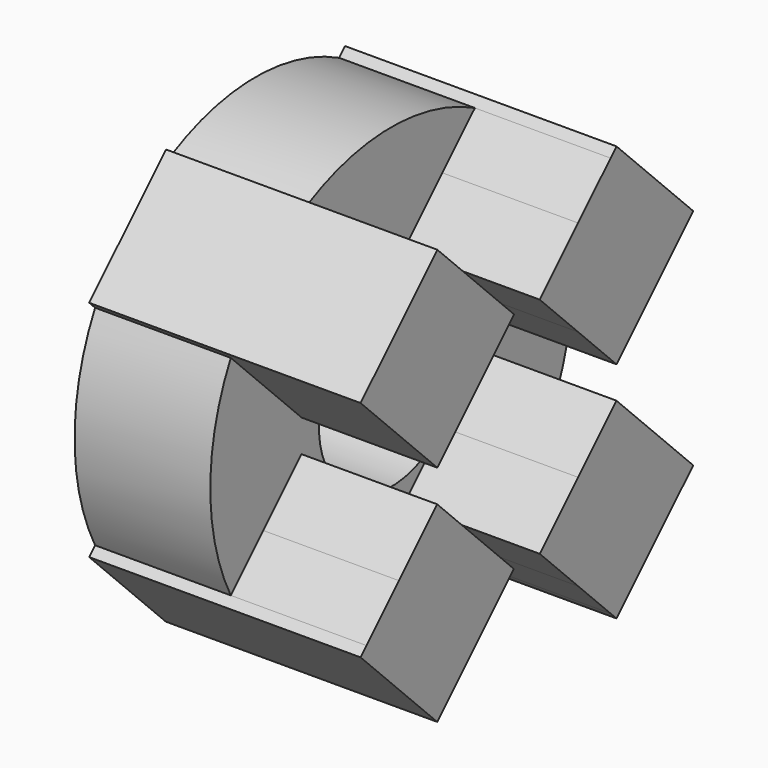
from build123d import *

# Parameters (mm, degrees)
F1_DEPTH = 7.62
F2_DEPTH = 15.24


with BuildPart() as f1:
    # F0 (on Right) → F1 (new body)
    with BuildSketch(Plane.YZ):
        with BuildLine():
            ThreePointArc((-22.7695842606, 19.3196809519), (-21.6955753206, 22.1687878641), (-21.330579045, 25.1916479534))
            ThreePointArc((-21.330579045, 25.1916479534), (-21.6955753206, 28.2145080427), (-22.7695842606, 31.063614955))
            Line((-22.7695842606, 31.063614955), (-25.0498647737, 28.7835671044))
            Line((-25.0498647737, 28.7835671044), (-25.0498647737, 21.5997288025))
            Line((-25.0498647737, 21.5997288025), (-22.7695842606, 19.3196809519))
        make_face()
        with BuildLine():
            Line((-25.0498647737, 28.7835671044), (-22.7695842606, 31.063614955))
            ThreePointArc((-22.7695842606, 31.063614955), (-23.7911283922, 32.7045468833), (-25.0498647737, 34.1714459009))
            Line((-25.0498647737, 34.1714459009), (-25.0498647737, 28.7835671044))
        make_face()
        with BuildLine():
            ThreePointArc((-24.8535283353, 16.4125967363), (-23.7086988595, 17.7924054626), (-22.7695842606, 19.3196809519))
            Line((-22.7695842606, 19.3196809519), (-25.0498647737, 21.5997288025))
            Line((-25.0498647737, 21.5997288025), (-25.0498647737, 16.2165853811))
            Line((-25.0498647737, 16.2165853811), (-24.8535283353, 16.4125967363))
        make_face()
        with BuildLine():
            Line((-30.4382933645, 34.1714459009), (-25.0498647737, 34.1714459009))
            ThreePointArc((-25.0498647737, 34.1714459009), (-26.5166353453, 35.4303319547), (-28.1574630291, 36.4520435177))
            Line((-28.1574630291, 36.4520435177), (-30.4382933645, 34.1714459009))
        make_face()
        Polygon((-25.0498647737, 28.7835671044), (-25.0498647737, 34.1714459009), (-30.4382933645, 34.1714459009), (-33.1322327207, 31.4777814138), (-30.4382933285, 28.7835671244), (-27.7443539522, 26.089352851), align=None)
        with BuildLine():
            Line((-25.0498647737, 21.5997288025), (-25.0498647737, 28.7835671044))
            Line((-25.0498647737, 28.7835671044), (-27.7443539522, 26.089352851))
            Line((-27.7443539522, 26.089352851), (-30.4382933285, 28.7835671244))
            ThreePointArc((-30.4382933285, 28.7835671244), (-29.3372214281, 27.1355600605), (-28.950579045, 25.1916479534))
            ThreePointArc((-28.950579045, 25.1916479534), (-29.3372214494, 23.2477357949), (-30.4382934071, 21.5997287037))
            Line((-30.4382934071, 21.5997287037), (-27.7443539522, 24.2939430558))
            Line((-27.7443539522, 24.2939430558), (-25.0498647737, 21.5997288025))
        make_face()
        Polygon((-25.0498647737, 16.2165853811), (-25.0498647737, 21.5997288025), (-27.7443539522, 24.2939430558), (-30.4382934071, 21.5997287037), (-33.1280466566, 18.9097009843), (-30.4299203819, 16.2118500059), (-25.0546080025, 16.2118500059), align=None)
        with BuildLine():
            Line((-30.4382933645, 34.1714459009), (-28.1574630291, 36.4520435177))
            ThreePointArc((-28.1574630291, 36.4520435177), (-34.0306965605, 37.8916479529), (-39.9039034491, 36.4519348256))
            Line((-39.9039034491, 36.4519348256), (-37.6234145244, 34.1714459009))
            Line((-37.6234145244, 34.1714459009), (-30.4382933645, 34.1714459009))
        make_face()
        with BuildLine():
            Line((-33.1322327207, 31.4777814138), (-30.4382933645, 34.1714459009))
            Line((-30.4382933645, 34.1714459009), (-37.6234145244, 34.1714459009))
            Line((-37.6234145244, 34.1714459009), (-34.9292002593, 31.4772316359))
            Line((-34.9292002593, 31.4772316359), (-37.6226815049, 28.7837503904))
            ThreePointArc((-37.6226815049, 28.7837503904), (-34.0304494597, 30.2716479518), (-30.4382933285, 28.7835671244))
            Line((-30.4382933285, 28.7835671244), (-33.1322327207, 31.4777814138))
        make_face()
        with BuildLine():
            Line((-37.6234145244, 34.1714459009), (-39.9039034491, 36.4519348256))
            ThreePointArc((-39.9039034491, 36.4519348256), (-41.5446174849, 35.4302624263), (-43.0112933162, 34.1714459009))
            Line((-43.0112933162, 34.1714459009), (-37.6234145244, 34.1714459009))
        make_face()
        Polygon((-34.9292002593, 31.4772316359), (-37.6234145244, 34.1714459009), (-43.0112933162, 34.1714459009), (-43.0112933162, 28.7830173475), (-40.317353932, 26.0890779633), (-37.6226815049, 28.7837503904), align=None)
        with BuildLine():
            ThreePointArc((-28.1519614983, 13.9341235479), (-26.6368414576, 14.865823798), (-25.2667473216, 16.0000619355))
            Line((-25.2667473216, 16.0000619355), (-25.0546080025, 16.2118500059))
            Line((-25.0546080025, 16.2118500059), (-30.4299203819, 16.2118500059))
            Line((-30.4299203819, 16.2118500059), (-28.1519614983, 13.9341235479))
        make_face()
        with BuildLine():
            Line((-33.1280466566, 18.9097009843), (-30.4382934071, 21.5997287037))
            ThreePointArc((-30.4382934071, 21.5997287037), (-37.6225898895, 21.5994539034), (-37.6226815049, 28.7837503904))
            Line((-37.6226815049, 28.7837503904), (-40.317353932, 26.0890779633))
            Line((-40.317353932, 26.0890779633), (-43.0112933162, 28.7830173475))
            Line((-43.0112933162, 28.7830173475), (-43.0112933162, 21.6024270559))
            Line((-43.0112933162, 21.6024270559), (-40.3278979877, 24.2860962057))
            Line((-40.3278979877, 24.2860962057), (-34.9473170757, 18.9060642873))
            Line((-34.9473170757, 18.9060642873), (-37.64125646, 16.2118500059))
            Line((-37.64125646, 16.2118500059), (-30.4299203819, 16.2118500059))
            Line((-30.4299203819, 16.2118500059), (-33.1280466566, 18.9097009843))
        make_face()
        with BuildLine():
            Line((-43.0112933162, 28.7830173475), (-43.0112933162, 34.1714459009))
            ThreePointArc((-43.0112933162, 34.1714459009), (-44.2700992213, 32.7044521275), (-45.2916825052, 31.0634065365))
            Line((-45.2916825052, 31.0634065365), (-43.0112933162, 28.7830173475))
        make_face()
        with BuildLine():
            ThreePointArc((-39.9154717637, 13.9374026349), (-34.034119179, 12.4916484468), (-28.1519614983, 13.9341235479))
            Line((-28.1519614983, 13.9341235479), (-30.4299203819, 16.2118500059))
            Line((-30.4299203819, 16.2118500059), (-37.64125646, 16.2118500059))
            Line((-37.64125646, 16.2118500059), (-39.9154717637, 13.9374026349))
        make_face()
        with BuildLine():
            Line((-43.0112933162, 28.7830173475), (-45.2916825052, 31.0634065365))
            ThreePointArc((-45.2916825052, 31.0634065365), (-46.7305790251, 25.1923579991), (-45.2923390044, 19.3211486035))
            Line((-45.2923390044, 19.3211486035), (-43.0112933162, 21.6024270559))
            Line((-43.0112933162, 21.6024270559), (-43.0112933162, 28.7830173475))
        make_face()
        with BuildLine():
            Line((-40.3262748881, 13.526557591), (-39.9154717637, 13.9374026349))
            ThreePointArc((-39.9154717637, 13.9374026349), (-41.5498772506, 14.9568956607), (-43.0112933162, 16.2118500059))
            ThreePointArc((-43.0112933162, 16.2118500059), (-44.2705192395, 17.6794162735), (-45.2923390044, 19.3211486035))
            Line((-45.2923390044, 19.3211486035), (-45.7073809685, 18.9060642873))
            Line((-45.7073809685, 18.9060642873), (-40.3262748881, 13.526557591))
        make_face()
        with BuildLine():
            ThreePointArc((-43.0112933162, 16.2118500059), (-41.5498772506, 14.9568956607), (-39.9154717637, 13.9374026349))
            Line((-39.9154717637, 13.9374026349), (-37.64125646, 16.2118500059))
            Line((-37.64125646, 16.2118500059), (-43.0112933162, 16.2118500059))
        make_face()
        Polygon((-43.0112933162, 16.2118500059), (-37.64125646, 16.2118500059), (-34.9473170757, 18.9060642873), (-40.3278979877, 24.2860962057), (-43.0112933162, 21.6024270559), align=None)
        with BuildLine():
            Line((-43.0112933162, 21.6024270559), (-45.2923390044, 19.3211486035))
            ThreePointArc((-45.2923390044, 19.3211486035), (-44.2705192395, 17.6794162735), (-43.0112933162, 16.2118500059))
            Line((-43.0112933162, 16.2118500059), (-43.0112933162, 21.6024270559))
        make_face()
    extrude(amount=F1_DEPTH)

    # F0 (on Right) → F2 (join)
    with BuildSketch(Plane.YZ):
        with BuildLine():
            Line((-25.0498647737, 28.7835671044), (-22.7695842606, 31.063614955))
            ThreePointArc((-22.7695842606, 31.063614955), (-23.7911283922, 32.7045468833), (-25.0498647737, 34.1714459009))
            Line((-25.0498647737, 34.1714459009), (-25.0498647737, 28.7835671044))
        make_face()
        with BuildLine():
            ThreePointArc((-25.0498647737, 34.1714459009), (-23.7911283922, 32.7045468833), (-22.7695842606, 31.063614955))
            Line((-22.7695842606, 31.063614955), (-22.3559253895, 31.4772316195))
            Line((-22.3559253895, 31.4772316195), (-25.0498647737, 34.1714459009))
        make_face()
        with BuildLine():
            Line((-22.3559253895, 18.9060642873), (-22.7695842606, 19.3196809519))
            ThreePointArc((-22.7695842606, 19.3196809519), (-23.7086988595, 17.7924054626), (-24.8535283353, 16.4125967363))
            Line((-24.8535283353, 16.4125967363), (-22.3559253895, 18.9060642873))
        make_face()
        with BuildLine():
            ThreePointArc((-24.8535283353, 16.4125967363), (-23.7086988595, 17.7924054626), (-22.7695842606, 19.3196809519))
            Line((-22.7695842606, 19.3196809519), (-25.0498647737, 21.5997288025))
            Line((-25.0498647737, 21.5997288025), (-25.0498647737, 16.2165853811))
            Line((-25.0498647737, 16.2165853811), (-24.8535283353, 16.4125967363))
        make_face()
        with BuildLine():
            Line((-30.4382933645, 34.1714459009), (-25.0498647737, 34.1714459009))
            ThreePointArc((-25.0498647737, 34.1714459009), (-26.5166353453, 35.4303319547), (-28.1574630291, 36.4520435177))
            Line((-28.1574630291, 36.4520435177), (-30.4382933645, 34.1714459009))
        make_face()
        Polygon((-25.0498647737, 28.7835671044), (-25.0498647737, 34.1714459009), (-30.4382933645, 34.1714459009), (-33.1322327207, 31.4777814138), (-30.4382933285, 28.7835671244), (-27.7443539522, 26.089352851), align=None)
        with BuildLine():
            ThreePointArc((-28.1574630291, 36.4520435177), (-26.5166353453, 35.4303319547), (-25.0498647737, 34.1714459009))
            Line((-25.0498647737, 34.1714459009), (-27.743804158, 36.8656601823))
            Line((-27.743804158, 36.8656601823), (-28.1574630291, 36.4520435177))
        make_face()
        Polygon((-25.0498647737, 16.2165853811), (-25.0498647737, 21.5997288025), (-27.7443539522, 24.2939430558), (-30.4382934071, 21.5997287037), (-33.1280466566, 18.9097009843), (-30.4299203819, 16.2118500059), (-25.0546080025, 16.2118500059), align=None)
        with BuildLine():
            Line((-37.6234145244, 34.1714459009), (-39.9039034491, 36.4519348256))
            ThreePointArc((-39.9039034491, 36.4519348256), (-41.5446174849, 35.4302624263), (-43.0112933162, 34.1714459009))
            Line((-43.0112933162, 34.1714459009), (-37.6234145244, 34.1714459009))
        make_face()
        with BuildLine():
            ThreePointArc((-43.0112933162, 34.1714459009), (-41.5446174849, 35.4302624263), (-39.9039034491, 36.4519348256))
            Line((-39.9039034491, 36.4519348256), (-40.317353932, 36.8653853085))
            Line((-40.317353932, 36.8653853085), (-43.0112933279, 34.1714459126))
        make_face()
        Polygon((-34.9292002593, 31.4772316359), (-37.6234145244, 34.1714459009), (-43.0112933162, 34.1714459009), (-43.0112933162, 28.7830173475), (-40.317353932, 26.0890779633), (-37.6226815049, 28.7837503904), align=None)
        with BuildLine():
            Line((-27.7443539522, 13.526557591), (-25.2667473216, 16.0000619355))
            ThreePointArc((-25.2667473216, 16.0000619355), (-26.6368414576, 14.865823798), (-28.1519614983, 13.9341235479))
            Line((-28.1519614983, 13.9341235479), (-27.7443539522, 13.526557591))
        make_face()
        with BuildLine():
            ThreePointArc((-28.1519614983, 13.9341235479), (-26.6368414576, 14.865823798), (-25.2667473216, 16.0000619355))
            Line((-25.2667473216, 16.0000619355), (-25.0546080025, 16.2118500059))
            Line((-25.0546080025, 16.2118500059), (-30.4299203819, 16.2118500059))
            Line((-30.4299203819, 16.2118500059), (-28.1519614983, 13.9341235479))
        make_face()
        with BuildLine():
            Line((-43.0112933162, 28.7830173475), (-43.0112933162, 34.1714459009))
            ThreePointArc((-43.0112933162, 34.1714459009), (-44.2700992213, 32.7044521275), (-45.2916825052, 31.0634065365))
            Line((-45.2916825052, 31.0634065365), (-43.0112933162, 28.7830173475))
        make_face()
        with BuildLine():
            ThreePointArc((-45.2916825052, 31.0634065365), (-44.2700992213, 32.7044521275), (-43.0112933162, 34.1714459009))
            Line((-43.0112933279, 34.1714459126), (-45.7055076046, 31.4772316359))
            Line((-45.7055076046, 31.4772316359), (-45.2916825052, 31.0634065365))
        make_face()
        with BuildLine():
            Line((-40.3262748881, 13.526557591), (-39.9154717637, 13.9374026349))
            ThreePointArc((-39.9154717637, 13.9374026349), (-41.5498772506, 14.9568956607), (-43.0112933162, 16.2118500059))
            ThreePointArc((-43.0112933162, 16.2118500059), (-44.2705192395, 17.6794162735), (-45.2923390044, 19.3211486035))
            Line((-45.2923390044, 19.3211486035), (-45.7073809685, 18.9060642873))
            Line((-45.7073809685, 18.9060642873), (-40.3262748881, 13.526557591))
        make_face()
        with BuildLine():
            ThreePointArc((-43.0112933162, 16.2118500059), (-41.5498772506, 14.9568956607), (-39.9154717637, 13.9374026349))
            Line((-39.9154717637, 13.9374026349), (-37.64125646, 16.2118500059))
            Line((-37.64125646, 16.2118500059), (-43.0112933162, 16.2118500059))
        make_face()
        Polygon((-43.0112933162, 16.2118500059), (-37.64125646, 16.2118500059), (-34.9473170757, 18.9060642873), (-40.3278979877, 24.2860962057), (-43.0112933162, 21.6024270559), align=None)
        with BuildLine():
            Line((-43.0112933162, 21.6024270559), (-45.2923390044, 19.3211486035))
            ThreePointArc((-45.2923390044, 19.3211486035), (-44.2705192395, 17.6794162735), (-43.0112933162, 16.2118500059))
            Line((-43.0112933162, 16.2118500059), (-43.0112933162, 21.6024270559))
        make_face()
    extrude(amount=F2_DEPTH)


solid = f1.part
